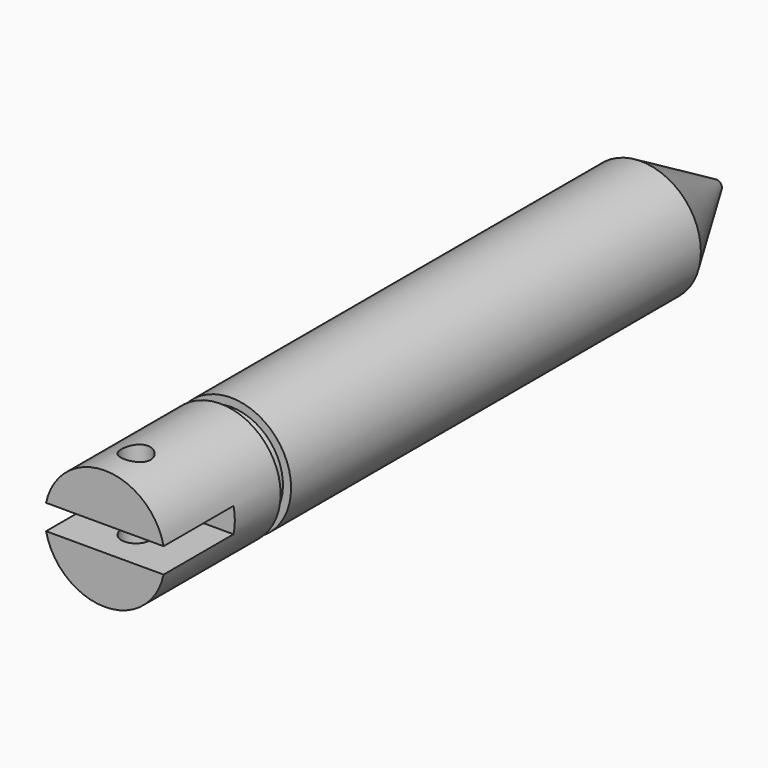
from build123d import *

# Parameters (mm, degrees)
F0_R     = 5.5
F1_DEPTH = 35
F2_SIZE2 = 8.6602540378
F2_SIZE  = 5
F4_W     = 13.5426148772
F4_H     = 2.286007395
F5_DEPTH = 8
F6_R     = 1.3316742147
F7_DEPTH = 10
F8_W     = 1.2
F8_H     = 1.4649596699
F8_H_2   = 0.745677419


with BuildPart() as f1:
    # F0 (on Front) → F1 (new body, symmetric)
    with BuildSketch(Plane.XZ):
        Circle(F0_R)
    extrude(amount=F1_DEPTH, both=True)

    # F2
    f2_edges = [f1.edges().sort_by_distance(p)[0] for p in [
        (-5.5, 35, 0),
    ]]
    f2_side = f1.faces().sort_by_distance((0, 35, 0))[0]
    chamfer(f2_edges, length=F2_SIZE, length2=F2_SIZE2, reference=f2_side)

    # F4 (on face) → F5 (cut)
    with BuildSketch(Plane.XZ.offset(35)):
        Rectangle(F4_W, F4_H)
    extrude(amount=-F5_DEPTH, mode=Mode.SUBTRACT)

    # F6 (on Top) → F7 (cut, symmetric)
    with BuildSketch(Plane.XY):
        with Locations((0, -31.4301326871)):
            Circle(F6_R)
    extrude(amount=F7_DEPTH, both=True, mode=Mode.SUBTRACT)

    # F8 (on Right) → F9 (revolve, cut)
    with BuildSketch(Plane.YZ):
        with Locations((-21.1584017664, 6.2324798349)):
            Rectangle(F8_W, F8_H)
        with Locations((-21.1584017664, 5.1271612905)):
            Rectangle(F8_W, F8_H_2)
    revolve(axis=Axis((0, -17.5, 0), (0, 1, 0)), mode=Mode.SUBTRACT)


with BuildPart() as f10_1:
    # F10: copy of F1
    add(f1.part.moved(Location((0, 0, 34))))


with BuildPart() as f12_1:
    # F12: copy of F1
    add(f1.part)


solid = f12_1.part
